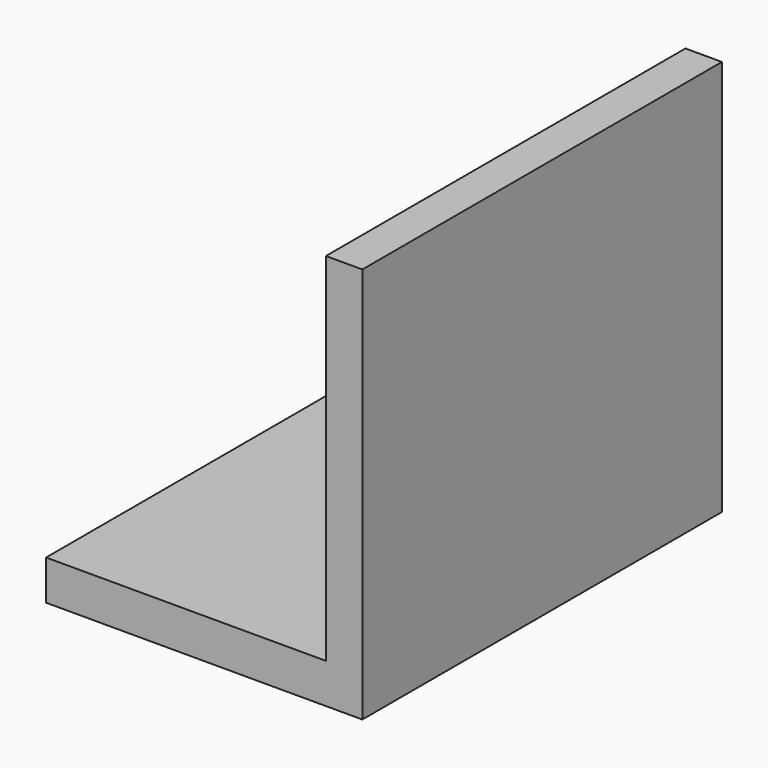
from build123d import *

# Parameters (mm, degrees)
F1_DEPTH = 80.625
F2_T     = -2.54


# Not quite as in the source:
# - a shell that OpenCascade refuses in one call is made with other operations: the cavity is built on its own and cut out


with BuildPart() as f1:
    # F0 (on Front) → F1 (new body)
    with BuildSketch(Plane.XZ):
        Polygon((0, 7.1409749798), (0, 0), (56.7328892648, 0), (56.7328892648, 71.0757300258), (50.1917116344, 71.0757300258), (50.1917116344, 7.1409749798), align=None)
    extrude(amount=F1_DEPTH)

    # F2: a shell. OpenCascade refuses it in one call, so the cavity is built on its own and cut out:
    # the body offset inwards by the wall thickness, plus a prism from it out through each open face.
    f2_core = offset(f1.part, amount=F2_T, kind=Kind.INTERSECTION, mode=Mode.PRIVATE)
    f2_exits = [f2_core.faces().sort_by_distance(p)[0] for p in [
        (52.731712, -40.3125, 36.568353),
    ]]
    add(f2_core, mode=Mode.SUBTRACT)
    extrude(f2_exits, amount=-F2_T, mode=Mode.SUBTRACT)


solid = f1.part
